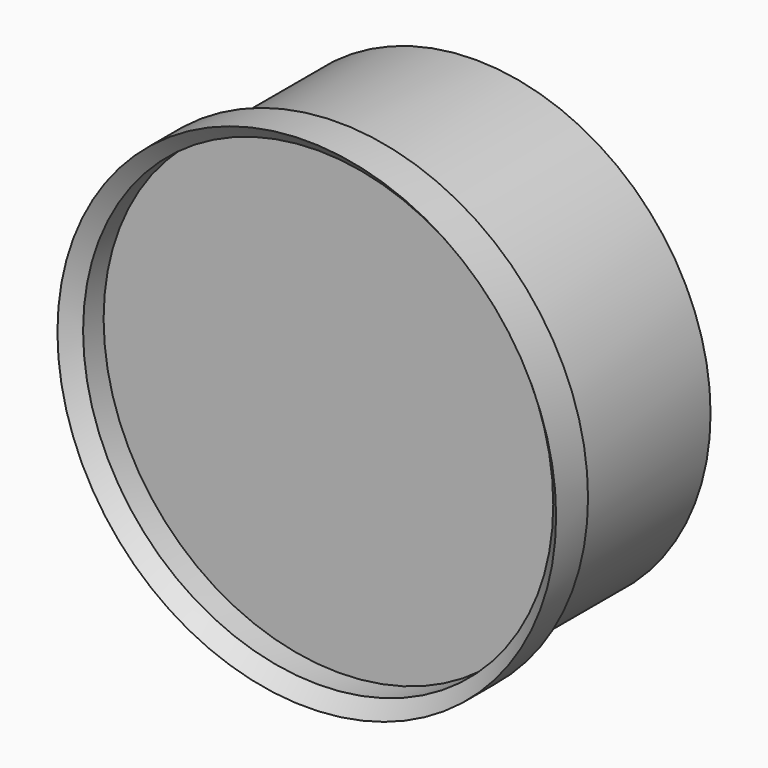
from build123d import *

# Parameters (mm, degrees)
F0_R     = 26.19375
F1_DEPTH = 19.05
F2_R     = 27.78125
F2_R_2   = 26.19375
F3_DEPTH = 7.9375


# Not quite as in the source:
# - a fillet or chamfer that OpenCascade refuses, or shapes differently, is made with other operations: its cross-section is extruded or revolved along the edge and cut away or added


with BuildPart() as f1:
    # F0 (on Front) → F1 (new body)
    with BuildSketch(Plane.XZ):
        Circle(F0_R)
    extrude(amount=F1_DEPTH)


with BuildPart() as f3:
    # F2 (on face) → F3 (new body)
    with BuildSketch(Plane.XZ.offset(19.05)):
        Circle(F2_R)
        Circle(F2_R_2, mode=Mode.SUBTRACT)
    extrude(amount=F3_DEPTH)

    # F4: chamfer of 5.08 on 1 edges, made by hand

    # F4_s1 → F4_t2 (revolve, cut)
    with BuildSketch(Plane.XY):
        Polygon((26.19375, -21.9075), (31.27375, -26.9875), (26.19375, -26.9875), align=None)
    revolve(axis=Axis((0, -26.9875, 0), (0, -1, 0)), mode=Mode.SUBTRACT)


solid = Compound([f1.part, f3.part])
